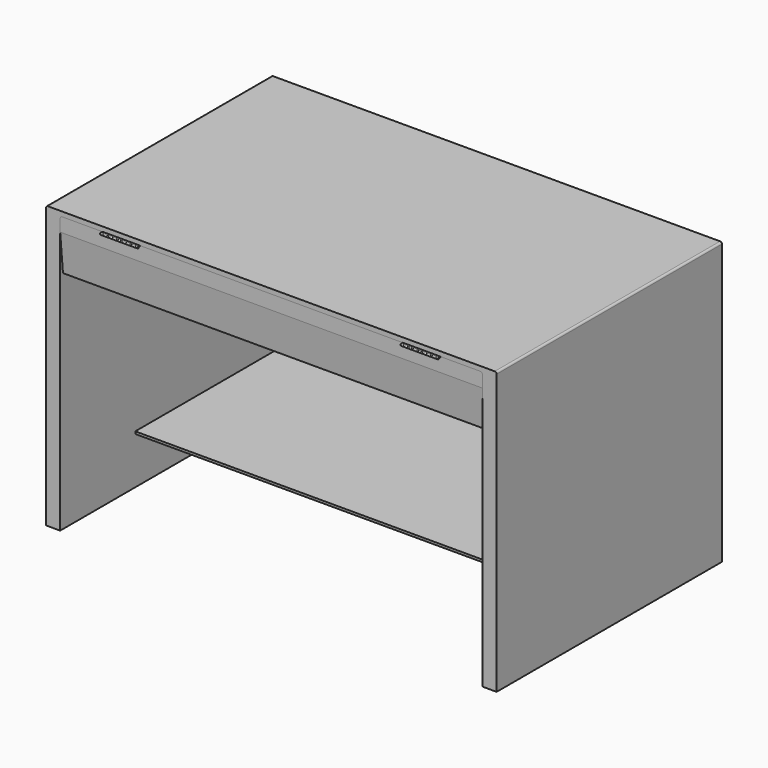
from build123d import *

# Parameters (mm, degrees)
F0_W      = 1143
F0_H      = 25.4
F0_H_2    = 228.6
F0_H_3    = 508
F1_DEPTH  = 38.1
F2_DEPTH  = 762
F3_SIZE   = 25.4
F4_R      = 5.08
F5_START  = -12.7
F5_DEPTH  = 139.7
F6_SIZE   = 25.39999
F7_R      = 5.08
F8_START  = -628.65
F8_DEPTH  = 6.35
F10_START = -152.4
F10_DEPTH = 101.6
F11_START = -965.2
F11_DEPTH = 101.6
F12_R     = 5.08
F13_R     = 5.08
F15_START = -50.8
F14_W     = 19.05
F14_H     = 692.15
F14_W_2   = 1104.9
F14_H_2   = 19.05
F15_DEPTH = 101.6
F16_START = -139.7
F16_DEPTH = 12.7
F17_SIZE2 = 9.525
F17_SIZE  = 101.6


# Not quite as in the source:
# - a fillet or chamfer is up to 0.001 mm smaller than in the source, because OpenCascade refuses the exact size


with BuildPart() as f1:
    # F0 (on Top) → F1 (new body)
    with BuildSketch(Plane.XY):
        with Locations((-571.5, -12.8375131965)):
            Rectangle(F0_W, F0_H)
        with Locations((-571.5, 114.1624868035)):
            Rectangle(F0_W, F0_H_2)
        with Locations((-571.5, 482.4624868035)):
            Rectangle(F0_W, F0_H_3)
    extrude(amount=-F1_DEPTH)

    # F0 (on Top) → F2 (join)
    with BuildSketch(Plane.XY):
        Polygon((-1143, 736.4624868035), (-1181.1, 736.4624868035), (-1181.1, -25.5375131965), (-1143, -25.5375131965), (-1143, -0.1375131965), (-1143, 228.4624868035), align=None)
        Polygon((38.1, 736.4624868035), (0, 736.4624868035), (0, 228.4624868035), (0, -0.1375131965), (0, -25.5375131965), (38.1, -25.5375131965), align=None)
    extrude(amount=-F2_DEPTH)

    # F3
    f3_edges = [f1.edges().sort_by_distance(p)[0] for p in [
        (-571.5, -25.537513, -38.1),
    ]]
    chamfer(f3_edges, length=F3_SIZE)

    # F4
    f4_edges = [f1.edges().sort_by_distance(p)[0] for p in [
        (-1143, -12.837513, -25.4),
        (0, -12.837513, -25.4),
    ]]
    fillet(f4_edges, radius=F4_R)

    # F12
    f12_edges = [f1.edges().sort_by_distance(p)[0] for p in [
        (-1181.1, 355.462487, 0),
    ]]
    fillet(f12_edges, radius=F12_R)

    # F13
    f13_edges = [f1.edges().sort_by_distance(p)[0] for p in [
        (38.1, 355.462487, 0),
    ]]
    fillet(f13_edges, radius=F13_R)


with BuildPart() as f5:
    # F0 (on Top) → F5 (new body)
    with BuildSketch(Plane.XY.offset(F5_START)):
        with Locations((-571.5, -12.8375131965)):
            Rectangle(F0_W, F0_H)
    extrude(amount=-F5_DEPTH)

    # F6 (size 25.4 in the source; OpenCascade refuses exactly that, so slightly less here)
    f6_edges = [f5.edges().sort_by_distance(p)[0] for p in [
        (-571.5, -0.137513, -12.7),
    ]]
    chamfer(f6_edges, length=F6_SIZE)

    # F7
    f7_edges = [f5.edges().sort_by_distance(p)[0] for p in [
        (-1143, -12.837508, -25.399995),
        (0, -12.837508, -25.399995),
    ]]
    fillet(f7_edges, radius=F7_R)

    # F17
    f17_edges = [f5.edges().sort_by_distance(p)[0] for p in [
        (-571.5, -25.537513, -152.4),
    ]]
    f17_side = f5.faces().sort_by_distance((-571.5, -25.537513, -82.556695))[0]
    chamfer(f17_edges, length=F17_SIZE, length2=F17_SIZE2, reference=f17_side)


with BuildPart() as f8:
    # F0 (on Top) → F8 (new body)
    with BuildSketch(Plane.XY.offset(F8_START)):
        with Locations((-571.5, 482.4624868035)):
            Rectangle(F0_W, F0_H_3)
    extrude(amount=-F8_DEPTH)


with BuildPart() as f10:
    # F9 (on face) → F10 (new body)
    with BuildSketch(Plane(origin=(-1181.1, 0, 0), x_dir=(0, -1, 0), z_dir=(-1, 0, 0)).offset(F10_START)):
        with BuildLine():
            ThreePointArc((29.6650131965, -14.9225), (33.4590580177, -16.4940448212), (31.8875131965, -12.7))
            Line((31.8875131965, -12.7), (31.8875131965, -14.9225))
            Line((31.8875131965, -14.9225), (29.6650131965, -14.9225))
        make_face()
        Polygon((31.8875131965, -12.7), (25.5375131965, -12.7), (25.5375131965, -14.9225), (29.6650131965, -14.9225), (31.8875131965, -14.9225), align=None)
        Polygon((25.5375131965, -14.9225), (23.3150131965, -14.9225), (0.1375131965, -38.1), (2.3600131965, -38.1), align=None)
        Polygon((25.5375131965, -14.9225), (25.5375131965, -12.7), (23.3150131965, -14.9225), align=None)
    extrude(amount=-F10_DEPTH)


with BuildPart() as f11:
    # F9 (on face) → F11 (new body)
    with BuildSketch(Plane(origin=(-1181.1, 0, 0), x_dir=(0, -1, 0), z_dir=(-1, 0, 0)).offset(F11_START)):
        Polygon((31.8875131965, -12.7), (25.5375131965, -12.7), (25.5375131965, -14.9225), (29.6650131965, -14.9225), (31.8875131965, -14.9225), align=None)
        with BuildLine():
            ThreePointArc((29.6650131965, -14.9225), (33.4590580177, -16.4940448212), (31.8875131965, -12.7))
            Line((31.8875131965, -12.7), (31.8875131965, -14.9225))
            Line((31.8875131965, -14.9225), (29.6650131965, -14.9225))
        make_face()
        Polygon((25.5375131965, -14.9225), (23.3150131965, -14.9225), (0.1375131965, -38.1), (2.3600131965, -38.1), align=None)
        Polygon((25.5375131965, -14.9225), (25.5375131965, -12.7), (23.3150131965, -14.9225), align=None)
    extrude(amount=-F11_DEPTH)


with BuildPart() as f15:
    # F14 (on face) → F15 (new body)
    with BuildSketch(Plane.XY.offset(F15_START)):
        with Locations((-1133.475, 345.9374868035)):
            Rectangle(F14_W, F14_H)
        with Locations((-9.525, 345.9374868035)):
            Rectangle(F14_W, F14_H)
        with Locations((-571.5, 701.5374868035)):
            Rectangle(F14_W_2, F14_H_2)
        with Locations((-9.525, 701.5374868035)):
            Rectangle(F14_W, F14_H_2)
        with Locations((-1133.475, 701.5374868035)):
            Rectangle(F14_W, F14_H_2)
    extrude(amount=-F15_DEPTH)

    # F14 (on face) → F16 (join)
    with BuildSketch(Plane.XY.offset(F16_START)):
        with Locations((-571.5, 345.9374868035)):
            Rectangle(F14_W_2, F14_H)
    extrude(amount=-F16_DEPTH)


solid = Compound([f1.part, f5.part, f8.part, f10.part, f11.part, f15.part])
